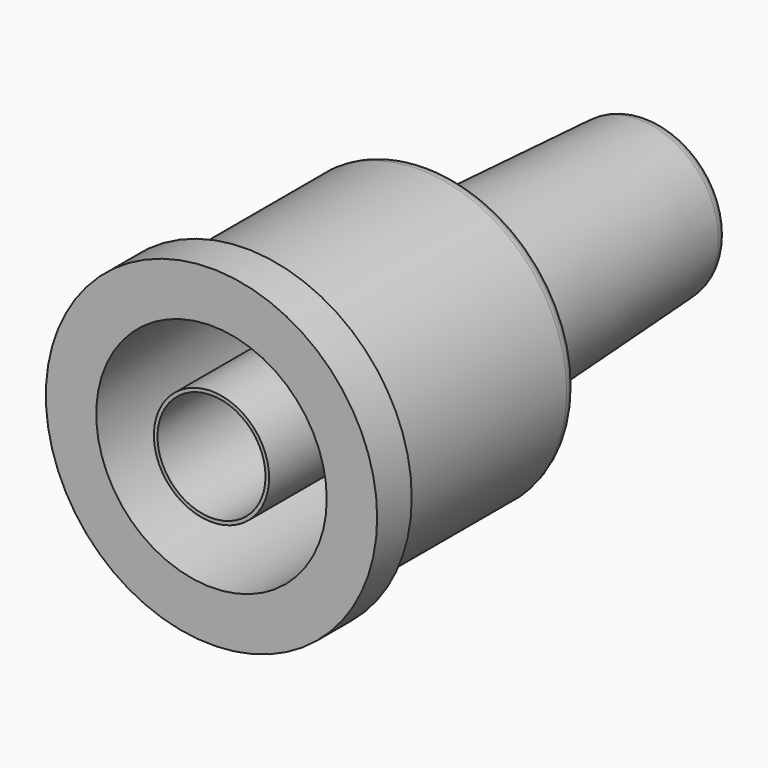
from build123d import *

# Parameters (mm, degrees)
F2_R      = 6.5
F0_R      = 5.5
F4_R      = 10.25
F5_DEPTH  = 19
F6_R      = 11.5
F7_DEPTH  = 3
F8_R      = 3.5
F9_DEPTH  = 19
F10_R     = 8
F11_DEPTH = 15
F12_R     = 4
F12_R_2   = 3.75
F13_DEPTH = 15
F14_R     = 1


with BuildPart() as f3:
    # F2 (on offset) → F3 section 0
    with BuildSketch(Plane.XZ.offset(19)):
        Circle(F2_R)
    # F0 (on Front) → F3 section 1
    with BuildSketch(Plane.XZ):
        Circle(F0_R)
    loft()

    # F4 (on face) → F5 (join)
    with BuildSketch(Plane.XZ.offset(19)):
        Circle(F4_R)
    extrude(amount=F5_DEPTH)

    # F6 (on face) → F7 (join)
    with BuildSketch(Plane.XZ.offset(38)):
        Circle(F6_R)
    extrude(amount=-F7_DEPTH)

    # F8 (on face) → F9 (cut)
    with BuildSketch(Plane(origin=(0, 0, 0), x_dir=(-1, 0, 0), z_dir=(0, 1, 0))):
        Circle(F8_R)
    extrude(amount=-F9_DEPTH, mode=Mode.SUBTRACT)

    # F10 (on face) → F11 (cut)
    with BuildSketch(Plane.XZ.offset(38)):
        Circle(F10_R)
    extrude(amount=-F11_DEPTH, mode=Mode.SUBTRACT)

    # F14
    f14_edges = [f3.edges().sort_by_distance(p)[0] for p in [
        (-5.5, 0, 0),
        (-10.25, -19, 0),
        (-6.5, -19, 0),
    ]]
    fillet(f14_edges, radius=F14_R)


with BuildPart() as f13:
    # F12 (on face) → F13 (new body)
    with BuildSketch(Plane.XZ.offset(23)):
        Circle(F12_R)
        Circle(F12_R_2, mode=Mode.SUBTRACT)
    extrude(amount=F13_DEPTH)


solid = Compound([f3.part, f13.part])
